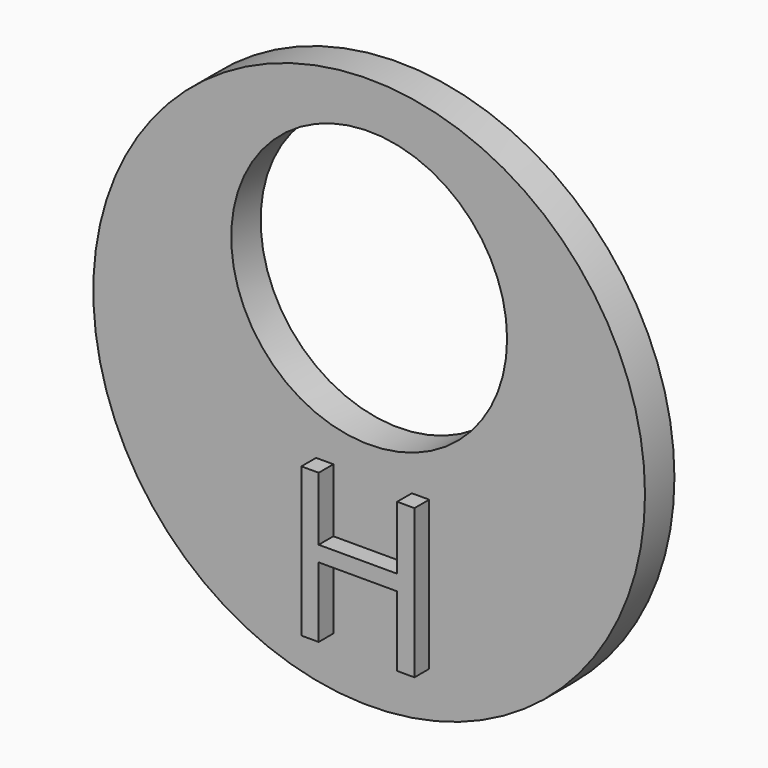
from build123d import *

# Parameters (mm, degrees)
F0_R         = 15
F0_R_2       = 7.5
F1_DEPTH     = 2
F2_TEXT_SIZE = 11.3475177305
F3_DEPTH     = 1


# Not quite as in the source:
# - Text() gives the source's letters only with a copy of the font that has no kerning and outlines rounded to 1/6400 em; it was checked with that copy


with BuildPart() as f1:
    # F0 (on Front) → F1 (new body)
    with BuildSketch(Plane.XZ):
        Circle(F0_R)
        with Locations((0, 5)):
            Circle(F0_R_2, mode=Mode.SUBTRACT)
    extrude(amount=F1_DEPTH)

    # F2 (on face) → F3 (join)
    with BuildSketch(Plane.XZ.offset(2)):
        with Locations((-4, -12.170212766)):
            Text('H', F2_TEXT_SIZE, font='Open Sans', text_align=(TextAlign.LEFT, TextAlign.BOTTOM))
    extrude(amount=F3_DEPTH)


solid = f1.part
